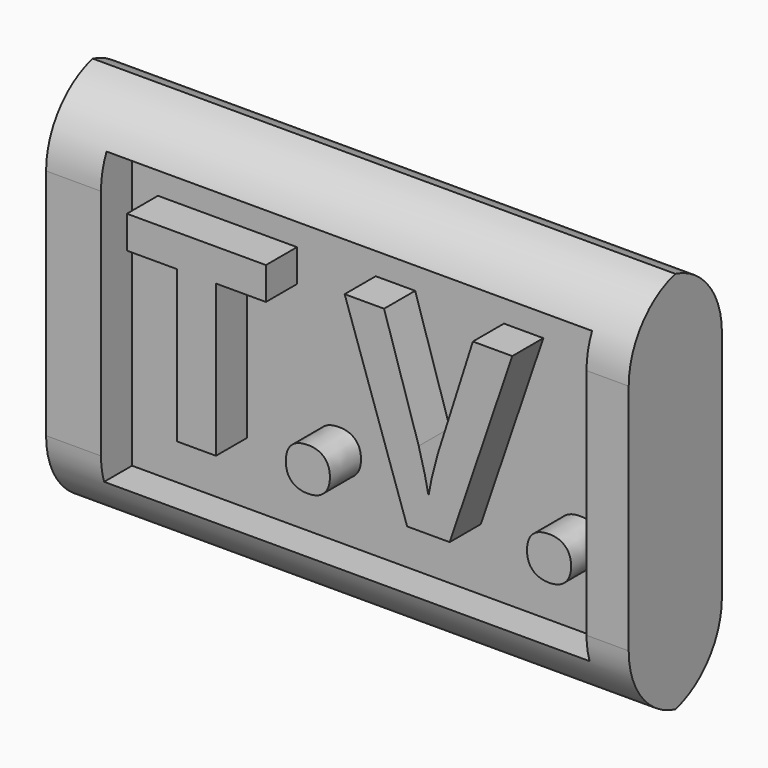
from build123d import *

# Parameters (mm, degrees)
F0_W         = 38.1
F0_H         = 25.4
F1_DEPTH     = 7.62
F2_W         = 31.7505737767
F2_H         = 18.9357784111
F3_DEPTH     = 2.54
F4_T1_DEPTH  = 63.5
F5_TEXT_SIZE = 16.8689034936
F6_DEPTH     = 2.54


# Not quite as in the source:
# - a fillet or chamfer that OpenCascade refuses, or shapes differently, is made with other operations: its cross-section is extruded or revolved along the edge and cut away or added
# - Text() gives the source's letters only with a copy of the font that has no kerning and outlines rounded to 1/6400 em; it was checked with that copy


with BuildPart() as f1:
    # F0 (on Front) → F1 (new body)
    with BuildSketch(Plane.XZ):
        with Locations((19.05, -12.7)):
            Rectangle(F0_W, F0_H)
    extrude(amount=F1_DEPTH)

    # F2 (on face) → F3 (cut)
    with BuildSketch(Plane.XZ.offset(7.62)):
        with Locations((19.4651898928, -12.4472355237)):
            Rectangle(F2_W, F2_H)
    extrude(amount=-F3_DEPTH, mode=Mode.SUBTRACT)

    # F4: fillet of radius 5.08 on 4 edges, made by hand

    # F4_s2 → F4_t1 (cut)
    with BuildSketch(Plane.YZ.offset(-12.7)):
        with BuildLine():
            ThreePointArc((-2.54, 0), (-6.1321024484, -1.4878975516), (-7.62, -5.08))
            Line((-7.62, -5.08), (-7.62, 0))
            Line((-7.62, 0), (-2.54, 0))
        make_face()
        with BuildLine():
            ThreePointArc((-5.08, 0), (-1.4878975516, -1.4878975516), (0, -5.08))
            Line((0, -5.08), (0, 0))
            Line((0, 0), (-5.08, 0))
        make_face()
        with BuildLine():
            ThreePointArc((-7.62, -20.32), (-6.1321024484, -23.9121024484), (-2.54, -25.4))
            Line((-2.54, -25.4), (-7.62, -25.4))
            Line((-7.62, -25.4), (-7.62, -20.32))
        make_face()
        with BuildLine():
            ThreePointArc((0, -20.32), (-1.4878975516, -23.9121024484), (-5.08, -25.4))
            Line((-5.08, -25.4), (0, -25.4))
            Line((0, -25.4), (0, -20.32))
        make_face()
    extrude(amount=F4_T1_DEPTH, mode=Mode.SUBTRACT)

    # F5 (on face) → F6 (join)
    with BuildSketch(Plane.XZ.offset(5.08)):
        with Locations((4.9461387349, -17.8670929984)):
            Text('T.V.', F5_TEXT_SIZE, font='Open Sans', font_style=FontStyle.BOLD, text_align=(TextAlign.LEFT, TextAlign.BOTTOM))
    extrude(amount=F6_DEPTH)


solid = f1.part
